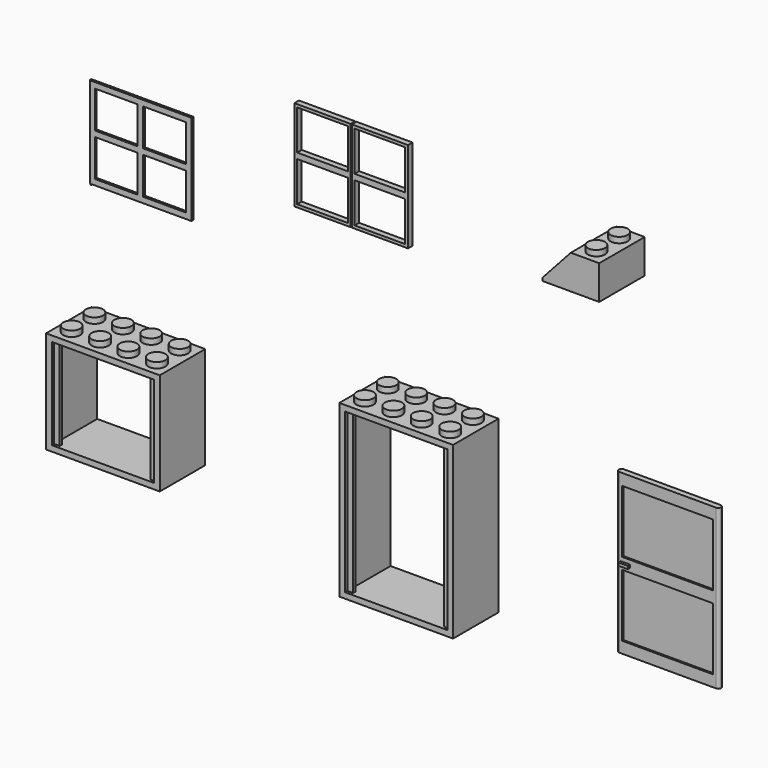
from build123d import *

# Parameters (mm, degrees)
F0_W          = 31.75
F0_H          = 47.625
F0_W_2        = 28.575
F0_H_2        = 44.45
F1_DEPTH      = 15.875
F0_H_3        = 28.575
F0_H_4        = 25.4
F2_DEPTH      = 15.875
F4_DEPTH      = 1.5875
F5_W          = 1.5875
F5_H          = 0.79502
F6_DEPTH      = 44.45
F7_D          = 0.3175
F7_DEPTH      = 0.3175
F7_TIP        = 0.0953866233
F0_W_3        = 25.4
F0_H_5        = 17.4625
F8_DEPTH      = 0.79502
F9_DEPTH      = 0.79502
F10_DEPTH     = 0.3175
F11_DEPTH     = 0.3175
F12_W         = 2.6039108634
F12_H         = 0.817257911
F13_DEPTH     = 0.79502
F14_W         = 1.5703439713
F14_H         = 0.6004769821
F15_DEPTH     = 0.79502
F16_R         = 0.79501
F17_R         = 0.15875
F18_DEPTH     = 0.3175
F19_T3_DEPTH  = 48.4251
F19_T8_DEPTH  = 48.4251
F19_T13_DEPTH = 48.4251
F19_T19_DEPTH = 48.4251
F19_T24_DEPTH = 48.4251
F19_T29_DEPTH = 48.4251
F20_R         = 2.38125
F21_DEPTH     = 1.5875
F22_W         = 1.5875
F22_H         = 0.79375
F23_DEPTH     = 25.4
F24_D         = 0.3175
F24_DEPTH     = 0.3175
F24_TIP       = 0.0953866233
F0_W_4        = 14.12621
F0_H_6        = 11.11123
F25_DEPTH     = 0.79502
F26_DEPTH     = 0.79502
F27_DEPTH     = 0.79502
F28_R         = 0.15875
F29_DEPTH     = 0.3175
F30_DEPTH     = 0.3175
F31_DEPTH     = 15.875
F32_R         = 2.38125
F33_DEPTH     = 1.5875
F0_W_5        = 11.90625
F0_H_7        = 10.31875
F34_DEPTH     = 0.3175
F35_DEPTH     = 0.3175
F36_R         = 0.31749
F37_R         = 0.15875
F38_DEPTH     = 0.3175


# Not quite as in the source:
# - a fillet or chamfer that OpenCascade refuses, or shapes differently, is made with other operations: its cross-section is extruded or revolved along the edge and cut away or added
# - a fillet or chamfer is up to 0.001 mm smaller than in the source, because OpenCascade refuses the exact size


with BuildPart() as f1:
    # F0 (on Front) → F1 (new body)
    with BuildSketch(Plane.XZ):
        Rectangle(F0_W, F0_H)
        Rectangle(F0_W_2, F0_H_2, mode=Mode.SUBTRACT)
    extrude(amount=F1_DEPTH)

    # F3 (on face) → F4 (join)
    with BuildSketch(Plane.XY.offset(23.8125)):
        with BuildLine():
            ThreePointArc((-9.525, -3.9624), (-13.5900480227, -2.2786019773), (-11.90625, -6.34365))
            Line((-11.90625, -6.34365), (-11.90625, -3.9624))
            Line((-11.90625, -3.9624), (-9.525, -3.9624))
        make_face()
        with BuildLine():
            ThreePointArc((-11.90625, -9.53135), (-13.5900480227, -13.5963980227), (-9.525, -11.9126))
            Line((-9.525, -11.9126), (-11.90625, -11.9126))
            Line((-11.90625, -11.9126), (-11.90625, -9.53135))
        make_face()
        with BuildLine():
            Line((-11.90625, -3.9624), (-11.90625, -6.34365))
            ThreePointArc((-11.90625, -6.34365), (-10.2224519773, -5.6461980227), (-9.525, -3.9624))
            Line((-9.525, -3.9624), (-11.90625, -3.9624))
        make_face()
        with BuildLine():
            Line((-3.95605, -3.9624), (-3.95605, -6.34365))
            ThreePointArc((-3.95605, -6.34365), (-2.2722519773, -5.6461980227), (-1.5748, -3.9624))
            ThreePointArc((-1.5748, -3.9624), (-3.95605, -1.58115), (-6.3373, -3.9624))
            Line((-6.3373, -3.9624), (-3.95605, -3.9624))
        make_face()
        with BuildLine():
            Line((-3.95605, -11.9126), (-6.3373, -11.9126))
            ThreePointArc((-6.3373, -11.9126), (-3.95605, -14.29385), (-1.5748, -11.9126))
            ThreePointArc((-1.5748, -11.9126), (-2.2722519773, -10.2288019773), (-3.95605, -9.53135))
            Line((-3.95605, -9.53135), (-3.95605, -11.9126))
        make_face()
        with BuildLine():
            ThreePointArc((3.9497, -9.53135), (2.2659019773, -13.5963980227), (6.33095, -11.9126))
            Line((6.33095, -11.9126), (3.9497, -11.9126))
            Line((3.9497, -11.9126), (3.9497, -9.53135))
        make_face()
        with BuildLine():
            ThreePointArc((11.8999, -9.53135), (10.2161019773, -10.2288019773), (9.51865, -11.9126))
            Line((9.51865, -11.9126), (11.8999, -11.9126))
            Line((11.8999, -11.9126), (11.8999, -9.53135))
        make_face()
        with BuildLine():
            Line((11.8999, -11.9126), (9.51865, -11.9126))
            ThreePointArc((9.51865, -11.9126), (11.8999, -14.29385), (14.28115, -11.9126))
            ThreePointArc((14.28115, -11.9126), (13.5836980227, -10.2288019773), (11.8999, -9.53135))
            Line((11.8999, -9.53135), (11.8999, -11.9126))
        make_face()
        with BuildLine():
            Line((3.9497, -11.9126), (6.33095, -11.9126))
            ThreePointArc((6.33095, -11.9126), (5.6334980227, -10.2288019773), (3.9497, -9.53135))
            Line((3.9497, -9.53135), (3.9497, -11.9126))
        make_face()
        with BuildLine():
            ThreePointArc((6.33095, -3.9624), (2.2659019773, -2.2786019773), (3.9497, -6.34365))
            Line((3.9497, -6.34365), (3.9497, -3.9624))
            Line((3.9497, -3.9624), (6.33095, -3.9624))
        make_face()
        with BuildLine():
            ThreePointArc((9.51865, -3.9624), (10.2161019773, -5.6461980227), (11.8999, -6.34365))
            Line((11.8999, -6.34365), (11.8999, -3.9624))
            Line((11.8999, -3.9624), (9.51865, -3.9624))
        make_face()
        with BuildLine():
            Line((-11.90625, -11.9126), (-9.525, -11.9126))
            ThreePointArc((-9.525, -11.9126), (-10.2224519773, -10.2288019773), (-11.90625, -9.53135))
            Line((-11.90625, -9.53135), (-11.90625, -11.9126))
        make_face()
        with BuildLine():
            ThreePointArc((-3.95605, -9.53135), (-5.6398480227, -10.2288019773), (-6.3373, -11.9126))
            Line((-6.3373, -11.9126), (-3.95605, -11.9126))
            Line((-3.95605, -11.9126), (-3.95605, -9.53135))
        make_face()
        with BuildLine():
            ThreePointArc((-6.3373, -3.9624), (-5.6398480227, -5.6461980227), (-3.95605, -6.34365))
            Line((-3.95605, -6.34365), (-3.95605, -3.9624))
            Line((-3.95605, -3.9624), (-6.3373, -3.9624))
        make_face()
        with BuildLine():
            Line((11.8999, -3.9624), (11.8999, -6.34365))
            ThreePointArc((11.8999, -6.34365), (13.5836980227, -5.6461980227), (14.28115, -3.9624))
            ThreePointArc((14.28115, -3.9624), (11.8999, -1.58115), (9.51865, -3.9624))
            Line((9.51865, -3.9624), (11.8999, -3.9624))
        make_face()
        with BuildLine():
            Line((3.9497, -3.9624), (3.9497, -6.34365))
            ThreePointArc((3.9497, -6.34365), (5.6334980227, -5.6461980227), (6.33095, -3.9624))
            Line((6.33095, -3.9624), (3.9497, -3.9624))
        make_face()
    extrude(amount=F4_DEPTH)

    # F5 (on face) → F6 (join)
    with BuildSketch(Plane.XY.offset(-22.225)):
        with Locations((13.49375, -14.68247)):
            Rectangle(F5_W, F5_H)
        with Locations((-13.49375, -14.68247)):
            Rectangle(F5_W, F5_H)
    extrude(amount=F6_DEPTH)

    # F7 (one way)
    with BuildSketch(Plane.XY.offset(-22.225)):
        with Locations((-13.49248, -15.47749), (13.49248, -15.47749)):
            Circle(F7_D / 2)
    extrude(amount=-F7_DEPTH, mode=Mode.SUBTRACT)
    with Locations(Plane.XY.offset(-22.225)):
        with Locations((-13.49248, -15.47749), (13.49248, -15.47749)):
            with Locations((0, 0, -(F7_DEPTH + F7_TIP / 2))):  # 118° drill point
                Cone(0, F7_D / 2, F7_TIP, mode=Mode.SUBTRACT)


with BuildPart() as f2:
    # F0 (on Front) → F2 (new body)
    with BuildSketch(Plane.XZ):
        with Locations((-81.9084644318, 0)):
            Rectangle(F0_W, F0_H_3)
        with Locations((-81.9084644318, 0)):
            Rectangle(F0_W_2, F0_H_4, mode=Mode.SUBTRACT)
    extrude(amount=F2_DEPTH)

    # F20 (on face) → F21 (join)
    with BuildSketch(Plane.XY.offset(14.2875)):
        with Locations((-77.9587644318, -3.9624)):
            Circle(F20_R)
        with Locations((-85.8581644318, -11.9126)):
            Circle(F20_R)
        with Locations((-93.8083644318, -11.9126)):
            Circle(F20_R)
        with Locations((-85.8581644318, -3.9624)):
            Circle(F20_R)
        with Locations((-93.8083644318, -3.9624)):
            Circle(F20_R)
        with Locations((-77.9587644318, -11.9126)):
            Circle(F20_R)
        with Locations((-70.0085644318, -11.9126)):
            Circle(F20_R)
        with Locations((-70.0085644318, -3.9624)):
            Circle(F20_R)
    extrude(amount=F21_DEPTH)

    # F22 (on face) → F23 (join)
    with BuildSketch(Plane.XY.offset(-12.7)):
        with Locations((-68.4147144318, -14.684375)):
            Rectangle(F22_W, F22_H)
        with Locations((-95.4022144318, -14.684375)):
            Rectangle(F22_W, F22_H)
    extrude(amount=F23_DEPTH)

    # F24 (one way)
    with BuildSketch(Plane.XY.offset(-12.7)):
        with Locations((-68.4159844318, -15.46352), (-95.4009444318, -15.46352)):
            Circle(F24_D / 2)
    extrude(amount=-F24_DEPTH, mode=Mode.SUBTRACT)
    with Locations(Plane.XY.offset(-12.7)):
        with Locations((-68.4159844318, -15.46352), (-95.4009444318, -15.46352)):
            with Locations((0, 0, -(F24_DEPTH + F24_TIP / 2))):  # 118° drill point
                Cone(0, F24_D / 2, F24_TIP, mode=Mode.SUBTRACT)


with BuildPart() as f8:
    # F0 (on Front) → F8 (new body)
    with BuildSketch(Plane.XZ):
        with Locations((63.7495815754, 0)):
            Rectangle(F0_W_2, F0_H_2)
        with Locations((63.7495815754, -10.31875)):
            Rectangle(F0_W_3, F0_H_5, mode=Mode.SUBTRACT)
        with Locations((63.7495815754, 10.31875)):
            Rectangle(F0_W_3, F0_H_5, mode=Mode.SUBTRACT)
    extrude(amount=F8_DEPTH)

    # F0 (on Front) → F9 (join)
    with BuildSketch(Plane.XZ):
        with Locations((63.7495815754, 0)):
            Rectangle(F0_W_2, F0_H_2)
        with Locations((63.7495815754, -10.31875)):
            Rectangle(F0_W_3, F0_H_5, mode=Mode.SUBTRACT)
        with Locations((63.7495815754, 10.31875)):
            Rectangle(F0_W_3, F0_H_5, mode=Mode.SUBTRACT)
    extrude(amount=-F9_DEPTH)

    # F0 (on Front) → F10 (join)
    with BuildSketch(Plane.XZ):
        with Locations((63.7495815754, 10.31875)):
            Rectangle(F0_W_3, F0_H_5)
        with Locations((63.7495815754, -10.31875)):
            Rectangle(F0_W_3, F0_H_5)
    extrude(amount=F10_DEPTH)

    # F0 (on Front) → F11 (join)
    with BuildSketch(Plane.XZ):
        with Locations((63.7495815754, -10.31875)):
            Rectangle(F0_W_3, F0_H_5)
        with Locations((63.7495815754, 10.31875)):
            Rectangle(F0_W_3, F0_H_5)
    extrude(amount=-F11_DEPTH)

    # F12 (on face) → F13 (join)
    with BuildSketch(Plane.XZ.offset(0.79502)):
        with Locations((51.958501339, 0)):
            Rectangle(F12_W, F12_H)
    extrude(amount=F13_DEPTH)

    # F14 (on face) → F15 (join)
    with BuildSketch(Plane(origin=(0, 0.79502, 0), x_dir=(-1, 0, 0), z_dir=(0, 1, 0))):
        with Locations((-50.7181398571, 0)):
            Rectangle(F14_W, F14_H)
    extrude(amount=F15_DEPTH)

    # F16 (radius 0.79502 in the source; OpenCascade refuses exactly that, so slightly less here)
    f16_edges = [f8.edges().sort_by_distance(p)[0] for p in [
        (78.037082, -0.79502, 0),
        (78.037082, 0.79502, 0),
    ]]
    fillet(f16_edges, radius=F16_R)

    # F17 (on face) → F18 (join)
    with BuildSketch(Plane(origin=(0, 0, -22.225), x_dir=(1, 0, 0), z_dir=(0, 0, -1))):
        with Locations((77.2420615754, 0)):
            Circle(F17_R)
    extrude(amount=F18_DEPTH)

    # F19: fillet of radius 0.79502 on 2 edges, made by hand


with BuildPart() as f19_tool1:
    # F19_s2 → F19_t3 (new body)
    with BuildSketch(Plane.XY.offset(24.21255)):
        with BuildLine():
            ThreePointArc((49.4620815754, 0), (49.6949375422, 0.5621640332), (50.2571015754, 0.79502))
            Line((50.2571015754, 0.79502), (49.4620815754, 0.79502))
            Line((49.4620815754, 0.79502), (49.4620815754, 0))
        make_face()
    extrude(amount=-F19_T3_DEPTH)

    split(bisect_by=Plane.XY.offset(0.300238491), keep=Keep.TOP)

    split(bisect_by=Plane.YZ.offset(49.9329678714), keep=Keep.BOTTOM)


with BuildPart() as f19_tool6:
    # F19_s7 → F19_t8 (new body)
    with BuildSketch(Plane.XY.offset(24.21255)):
        with BuildLine():
            ThreePointArc((49.4620815754, 0), (49.6949375422, 0.5621640332), (50.2571015754, 0.79502))
            Line((50.2571015754, 0.79502), (49.4620815754, 0.79502))
            Line((49.4620815754, 0.79502), (49.4620815754, 0))
        make_face()
    extrude(amount=-F19_T8_DEPTH)

    split(bisect_by=Plane.XY.offset(0.300238491), keep=Keep.TOP)

    split(bisect_by=Plane.YZ.offset(49.9329678714), keep=Keep.TOP)


with BuildPart() as f19_tool11:
    # F19_s12 → F19_t13 (new body)
    with BuildSketch(Plane.XY.offset(24.21255)):
        with BuildLine():
            ThreePointArc((49.4620815754, 0), (49.6949375422, 0.5621640332), (50.2571015754, 0.79502))
            Line((50.2571015754, 0.79502), (49.4620815754, 0.79502))
            Line((49.4620815754, 0.79502), (49.4620815754, 0))
        make_face()
    extrude(amount=-F19_T13_DEPTH)

    split(bisect_by=Plane.XY.offset(0.300238491), keep=Keep.BOTTOM)

    split(bisect_by=Plane.YZ.offset(49.9329678714), keep=Keep.BOTTOM)

    split(bisect_by=Plane.XY.offset(-0.300238491), keep=Keep.TOP)


with BuildPart() as f19_tool17:
    # F19_s18 → F19_t19 (new body)
    with BuildSketch(Plane.XY.offset(24.21255)):
        with BuildLine():
            ThreePointArc((49.4620815754, 0), (49.6949375422, 0.5621640332), (50.2571015754, 0.79502))
            Line((50.2571015754, 0.79502), (49.4620815754, 0.79502))
            Line((49.4620815754, 0.79502), (49.4620815754, 0))
        make_face()
    extrude(amount=-F19_T19_DEPTH)

    split(bisect_by=Plane.YZ.offset(49.9329678714), keep=Keep.BOTTOM)

    split(bisect_by=Plane.XY.offset(-0.300238491), keep=Keep.BOTTOM)


with BuildPart() as f19_tool22:
    # F19_s23 → F19_t24 (new body)
    with BuildSketch(Plane.XY.offset(24.21255)):
        with BuildLine():
            ThreePointArc((49.4620815754, 0), (49.6949375422, 0.5621640332), (50.2571015754, 0.79502))
            Line((50.2571015754, 0.79502), (49.4620815754, 0.79502))
            Line((49.4620815754, 0.79502), (49.4620815754, 0))
        make_face()
    extrude(amount=-F19_T24_DEPTH)

    split(bisect_by=Plane.YZ.offset(49.9329678714), keep=Keep.TOP)

    split(bisect_by=Plane.XY.offset(-0.300238491), keep=Keep.BOTTOM)


with BuildPart() as f19_tool27:
    # F19_s28 → F19_t29 (new body)
    with BuildSketch(Plane.XY.offset(24.21255)):
        with BuildLine():
            ThreePointArc((50.2571015754, -0.79502), (49.6949375422, -0.5621640332), (49.4620815754, 0))
            Line((49.4620815754, 0), (49.4620815754, -0.79502))
            Line((49.4620815754, -0.79502), (50.2571015754, -0.79502))
        make_face()
    extrude(amount=-F19_T29_DEPTH)


with BuildPart() as f8_1:
    add(f8.part)

    # F19_t30: cut F19_tool1, F19_tool6, F19_tool11, F19_tool17, F19_tool22, F19_tool27
    add([f19_tool1.part, f19_tool6.part, f19_tool11.part, f19_tool17.part, f19_tool22.part, f19_tool27.part], mode=Mode.SUBTRACT)


with BuildPart() as f25:
    # F0 (on Front) → F25 (new body)
    with BuildSketch(Plane.XZ):
        Polygon((-24.4821571088, 57.976230979), (-8.7659071088, 57.976230979), (-8.7659071088, 69.882480979), (-8.7659071088, 71.469980979), (-8.7659071088, 83.376230979), (-24.4821571088, 83.376230979), align=None)
        with Locations((-16.6240321088, 64.326865979)):
            Rectangle(F0_W_4, F0_H_6, mode=Mode.SUBTRACT)
        with Locations((-16.6240321088, 77.025595979)):
            Rectangle(F0_W_4, F0_H_6, mode=Mode.SUBTRACT)
    extrude(amount=F25_DEPTH)

    # F0 (on Front) → F26 (join)
    with BuildSketch(Plane.XZ):
        Polygon((-24.4821571088, 57.976230979), (-8.7659071088, 57.976230979), (-8.7659071088, 69.882480979), (-8.7659071088, 71.469980979), (-8.7659071088, 83.376230979), (-24.4821571088, 83.376230979), align=None)
        with Locations((-16.6240321088, 64.326865979)):
            Rectangle(F0_W_4, F0_H_6, mode=Mode.SUBTRACT)
        with Locations((-16.6240321088, 77.025595979)):
            Rectangle(F0_W_4, F0_H_6, mode=Mode.SUBTRACT)
    extrude(amount=-F26_DEPTH)

    # F28 (on face) → F29 (join)
    with BuildSketch(Plane(origin=(0, 0, 57.976230979), x_dir=(1, 0, 0), z_dir=(0, 0, -1))):
        with Locations((-9.5529677346, 0)):
            Circle(F28_R)
    extrude(amount=F29_DEPTH)


with BuildPart() as f25b:
    # F0 (on Front) → F25, piece 2 (new body)
    with BuildSketch(Plane.XZ):
        Polygon((-40.5159071088, 69.882480979), (-40.5159071088, 57.976230979), (-24.7996571088, 57.976230979), (-24.7996571088, 83.376230979), (-40.5159071088, 83.376230979), (-40.5159071088, 71.469980979), align=None)
        with Locations((-32.6577821088, 64.326865979)):
            Rectangle(F0_W_4, F0_H_6, mode=Mode.SUBTRACT)
        with Locations((-32.6577821088, 77.025595979)):
            Rectangle(F0_W_4, F0_H_6, mode=Mode.SUBTRACT)
    extrude(amount=F25_DEPTH)

    # F0 (on Front) → F27 (join)
    with BuildSketch(Plane.XZ):
        Polygon((-40.5159071088, 69.882480979), (-40.5159071088, 57.976230979), (-24.7996571088, 57.976230979), (-24.7996571088, 83.376230979), (-40.5159071088, 83.376230979), (-40.5159071088, 71.469980979), align=None)
        with Locations((-32.6577821088, 64.326865979)):
            Rectangle(F0_W_4, F0_H_6, mode=Mode.SUBTRACT)
        with Locations((-32.6577821088, 77.025595979)):
            Rectangle(F0_W_4, F0_H_6, mode=Mode.SUBTRACT)
    extrude(amount=-F27_DEPTH)

    # F28 (on face) → F30 (join)
    with BuildSketch(Plane(origin=(0, 0, 57.976230979), x_dir=(1, 0, 0), z_dir=(0, 0, -1))):
        with Locations((-39.7183820605, 0)):
            Circle(F28_R)
    extrude(amount=F30_DEPTH)


with BuildPart() as f31:
    # F0 (on Front) → F31 (new body)
    with BuildSketch(Plane.XZ):
        Polygon((40.8194512129, 72.2287893295), (56.6944512129, 72.2287893295), (56.6944512129, 81.7537893295), (48.7569512129, 81.7537893295), (40.8194512129, 73.0238093295), align=None)
    extrude(amount=F31_DEPTH)

    # F32 (on face) → F33 (join)
    with BuildSketch(Plane.XY.offset(81.7537893295)):
        with Locations((52.7257012129, -11.9126)):
            Circle(F32_R)
        with Locations((52.7257012129, -3.9624)):
            Circle(F32_R)
    extrude(amount=F33_DEPTH)


with BuildPart() as f34:
    # F0 (on Front) → F34 (new body)
    with BuildSketch(Plane.XZ):
        with Locations((-83.8944480658, 57.4049114347)):
            Rectangle(F0_W_2, F0_H_4)
        with Locations((-90.6413230658, 51.4517864347)):
            Rectangle(F0_W_5, F0_H_7, mode=Mode.SUBTRACT)
        with Locations((-77.1475730658, 51.4517864347)):
            Rectangle(F0_W_5, F0_H_7, mode=Mode.SUBTRACT)
        with Locations((-90.6413230658, 63.3580364347)):
            Rectangle(F0_W_5, F0_H_7, mode=Mode.SUBTRACT)
        with Locations((-77.1475730658, 63.3580364347)):
            Rectangle(F0_W_5, F0_H_7, mode=Mode.SUBTRACT)
    extrude(amount=F34_DEPTH)

    # F0 (on Front) → F35 (join)
    with BuildSketch(Plane.XZ):
        with Locations((-83.8944480658, 57.4049114347)):
            Rectangle(F0_W_2, F0_H_4)
        with Locations((-90.6413230658, 51.4517864347)):
            Rectangle(F0_W_5, F0_H_7, mode=Mode.SUBTRACT)
        with Locations((-77.1475730658, 51.4517864347)):
            Rectangle(F0_W_5, F0_H_7, mode=Mode.SUBTRACT)
        with Locations((-90.6413230658, 63.3580364347)):
            Rectangle(F0_W_5, F0_H_7, mode=Mode.SUBTRACT)
        with Locations((-77.1475730658, 63.3580364347)):
            Rectangle(F0_W_5, F0_H_7, mode=Mode.SUBTRACT)
    extrude(amount=-F35_DEPTH)

    # F36 (radius 0.3175 in the source; OpenCascade refuses exactly that, so slightly less here)
    f36_edges = [f34.edges().sort_by_distance(p)[0] for p in [
        (-98.181948, -0.3175, 57.404911),
        (-98.181948, 0.3175, 57.404911),
    ]]
    fillet(f36_edges, radius=F36_R)

    # F37 (on face) → F38 (join)
    with BuildSketch(Plane(origin=(0, 0, 44.7049114347), x_dir=(1, 0, 0), z_dir=(0, 0, -1))):
        with Locations((-97.8644480658, 0)):
            Circle(F37_R)
    extrude(amount=F38_DEPTH)


solid = Compound([f1.part, f2.part, f8_1.part, f25.part, f25b.part, f31.part, f34.part])
